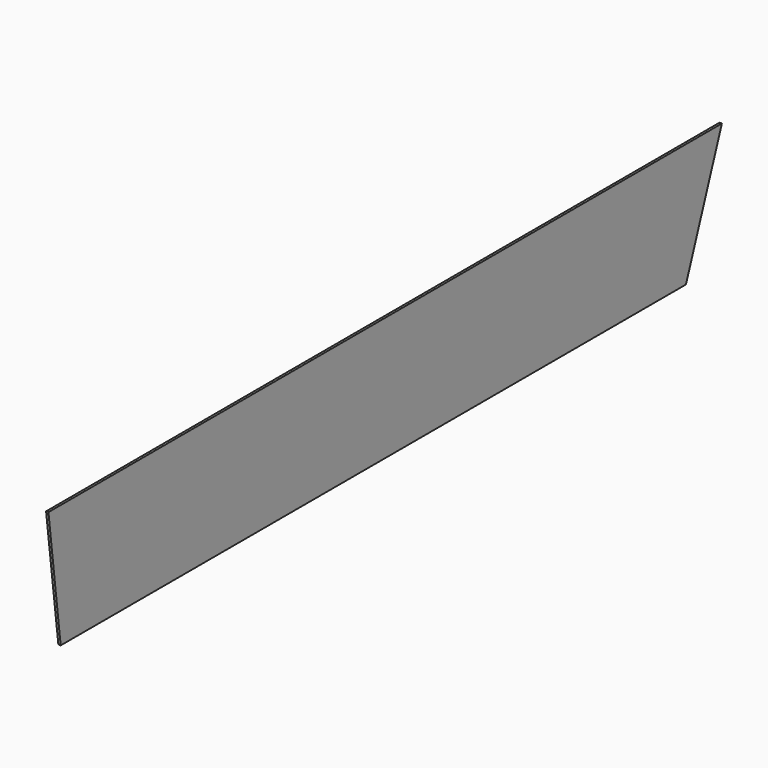
from build123d import *

# Parameters (mm, degrees)
F1_DEPTH = 4.7625


# Not quite as in the source:
# - a length typed as a fraction of an inch, garbled in the dataset ("3 / 203.2 mm" for 3/8 in), is restored


with BuildPart() as f1:
    # F0 (on Right) → F1 (new body)
    with BuildSketch(Plane.YZ):
        Polygon((-839.8578202019, 123.825), (-808.7468078986, -127), (778.2749994396, -127), (869.5678334494, 123.825), align=None)
    extrude(amount=F1_DEPTH)


solid = f1.part
